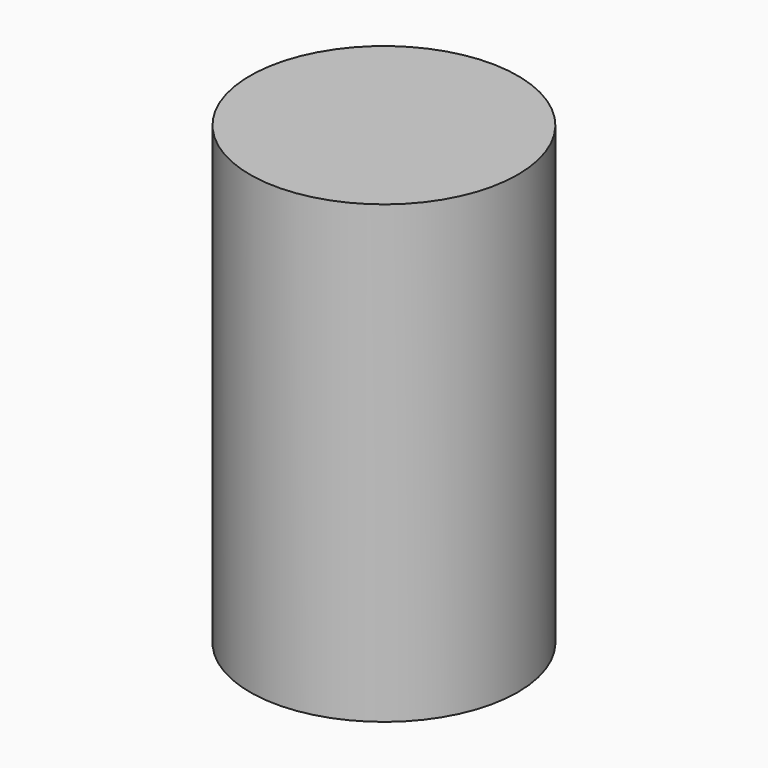
from build123d import *

# Parameters (mm, degrees)
F2_R     = 52.6346493219
F3_DEPTH = 179.07


# Not quite as in the source:
# - the program builds the solid bodies; features that only make, move or delete a surface that nothing else refers to are left out


with BuildPart() as f3:
    # F2 (on Top) → F3 (new body)
    with BuildSketch(Plane.XY):
        Circle(F2_R)
    extrude(amount=F3_DEPTH)


solid = f3.part
